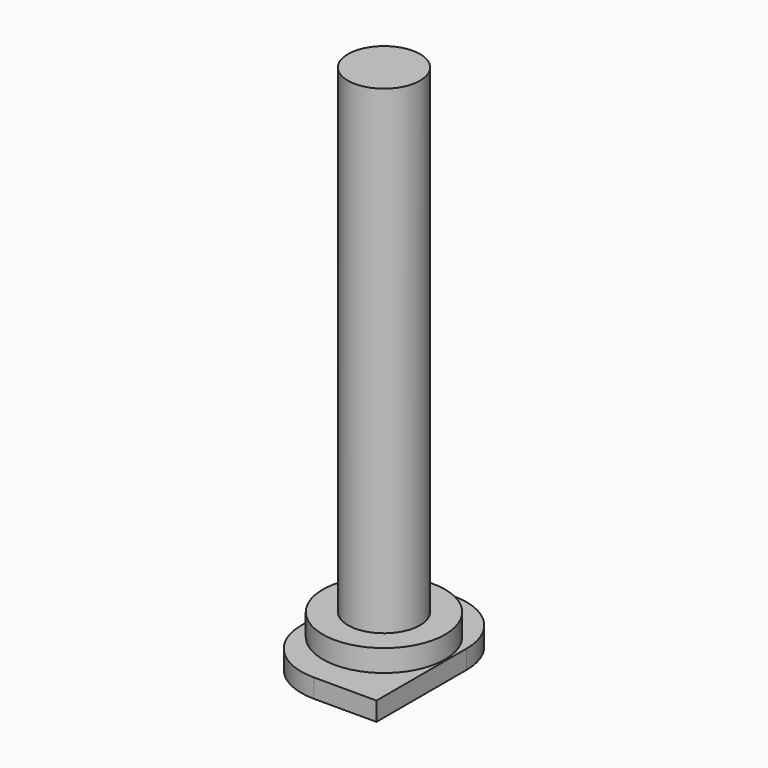
from build123d import *

# Parameters (mm, degrees)
F0_R     = 2.875
F1_DEPTH = 20
F2_W     = 10
F2_H     = 14
F2_R     = 2.875
F3_DEPTH = 1.5
F4_R     = 5
F5_R     = 4.875
F5_R_2   = 2.875
F6_DEPTH = 1.75


with BuildPart() as f1:
    # F0 (on Top) → F1 (new body, symmetric)
    with BuildSketch(Plane.XY):
        Circle(F0_R)
    extrude(amount=F1_DEPTH, both=True)

    # F2 (on face) → F3 (join)
    with BuildSketch(Plane(origin=(0, 0, -20), x_dir=(1, 0, 0), z_dir=(0, 0, -1))):
        Rectangle(F2_W, F2_H)
        Circle(F2_R, mode=Mode.SUBTRACT)
        Circle(F2_R)
    extrude(amount=F3_DEPTH)

    # F4
    f4_edges = [f1.edges().sort_by_distance(p)[0] for p in [
        (-5, -7, -20.75),
        (5, 7, -20.75),
    ]]
    fillet(f4_edges, radius=F4_R)

    # F5 (on face) → F6 (join)
    with BuildSketch(Plane.XY.offset(-20)):
        Circle(F5_R)
        Circle(F5_R_2, mode=Mode.SUBTRACT)
    extrude(amount=F6_DEPTH)


solid = f1.part
